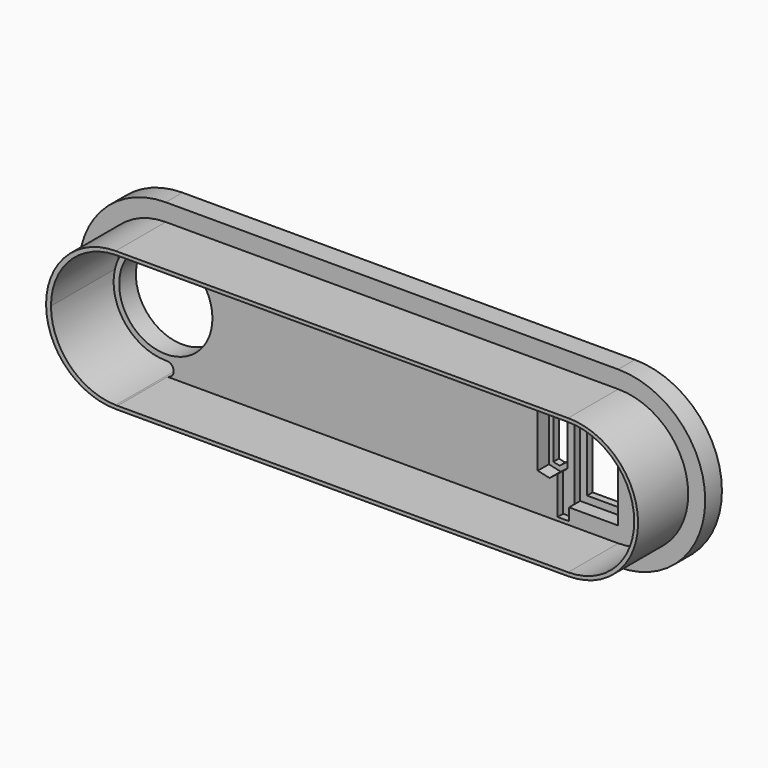
from build123d import *

# Parameters (mm, degrees)
F0_R     = 6.7
F1_DEPTH = 3
F2_DEPTH = 2
F0_W     = 5
F0_H     = 12.5
F3_DEPTH = 1
F4_DEPTH = 12


# Not quite as in the source:
# - ends of sketch curves that miss each other by under 0.0002 mm in the source are joined
# - a feature names something its author has since deleted; it is built from what else it names


with BuildPart() as f1:
    # F0 (on Front) → F1 (new body)
    with BuildSketch(Plane.XZ):
        with BuildLine():
            ThreePointArc((-65, 22), (-63.9934095883, 20.9934095883), (-65, 19.9868191765))
            ThreePointArc((-65, 19.9868191765), (-72.5, 12.4868191765), (-65, 4.9868191765))
            ThreePointArc((-65, 4.9868191765), (-63.8767141262, 4.1275392339), (-64.7360688632, 3.0043105795))
            Line((-64.7360688632, 3.0043105795), (0, 3))
            ThreePointArc((0, 3), (9.5, 12.5), (0, 22))
            Line((0, 22), (-65, 22))
        make_face()
        with Locations((-65, 12.4868191765)):
            Circle(F0_R, mode=Mode.SUBTRACT)
        Polygon((-7.0638221186, 19.7500795352), (-0.0638221186, 19.7500795352), (-0.0638221186, 5.2500795352), (-7.0638221186, 5.2500795352), (-7.0638221186, 3.5000024036), (-8.713822115, 3.5001122721), (-8.713822115, 8.9301122721), (-9.8584694148, 8.0498078222), (-11.5638221186, 8.4283766224), (-11.5638221186, 12.5000409694), (-11.5638221186, 16.5717053165), (-9.8584694148, 16.9502741166), (-8.713822115, 16.0699696667), (-8.713822115, 21.4999696667), (-7.0638221186, 21.5000795352), align=None, mode=Mode.SUBTRACT)
    extrude(amount=F1_DEPTH)



with BuildPart() as f1b:
    # F0 (on Front) → F1, piece 2 (new body)
    with BuildSketch(Plane.XZ):
        with BuildLine():
            Line((-65, 0), (0, 0))
            ThreePointArc((0, 0), (12.5, 12.5), (0, 25))
            Line((0, 25), (-65, 25))
            ThreePointArc((-65, 25), (-77.5, 12.5), (-65, 0))
        make_face()
        with BuildLine():
            ThreePointArc((-2.276e-07, 22.5000819376), (10.0557466602, 12.5000410832), (0, 2.5))
            Line((0, 2.5), (-65, 2.5))
            ThreePointArc((-65, 2.5), (-75.0000410826, 12.500040855), (-65.0000002276, 22.5000819376))
            Line((-65.0000002276, 22.5000819376), (-2.276e-07, 22.5000819376))
        make_face(mode=Mode.SUBTRACT)
    extrude(amount=F1_DEPTH)


with BuildPart() as f2:
    # F0 (on Front) → F2 (new body)
    with BuildSketch(Plane.XZ):
        Polygon((-7.0638221186, 12.5000795352), (-7.0638221186, 19.7500795352), (-7.0638221186, 21.5000795352), (-8.713822115, 21.4999696667), (-8.713822115, 16.0699696667), (-8.0638221186, 15.5700795352), (-8.0638221186, 9.4300024036), (-8.713822115, 8.9301122721), (-8.713822115, 3.5001122721), (-7.0638221186, 3.5000024036), (-7.0638221186, 5.2500024036), (-7.0638221186, 9.4300024036), align=None)
    extrude(amount=F2_DEPTH)


with BuildPart() as f3:
    # F0 (on Front) → F3 (new body)
    with BuildSketch(Plane.XZ):
        Polygon((-0.0638221186, 5.2500795352), (-0.0638221186, 19.7500795352), (-7.0638221186, 19.7500795352), (-7.0638221186, 12.5000795352), (-7.0638221186, 9.4300024036), (-7.0638221186, 5.2500795352), align=None)
        with Locations((-3.5638221186, 12.5000795352)):
            Rectangle(F0_W, F0_H, mode=Mode.SUBTRACT)
    extrude(amount=F3_DEPTH)


with BuildPart() as f3b:
    # F0 (on Front) → F3, piece 2 (new body)
    with BuildSketch(Plane.XZ):
        Polygon((-8.0638221186, 15.5700795352), (-8.713822115, 16.0699696667), (-9.8584694148, 16.9502741166), (-11.5638221186, 16.5717053165), (-11.5638221186, 12.5000409694), (-11.5638221186, 8.4283766224), (-9.8584694148, 8.0498078222), (-8.713822115, 8.9301122721), (-8.0638221186, 9.4300024036), align=None)
        Polygon((-10.0138316441, 16.249757261), (-8.7138221186, 15.2499696667), (-8.7138221186, 9.7501122721), (-10.0138316441, 8.7503246778), (-10.9138221186, 8.9501122721), (-10.9138221186, 9.7501122721), (-10.9138221186, 16.0499696667), align=None, mode=Mode.SUBTRACT)
    extrude(amount=F3_DEPTH)


with BuildPart() as f1_1:
    add(f1.part)

    add(f1b.part)  # F4 merges F1b
    # F0 (on Front) → F4 (join)
    with BuildSketch(Plane.XZ):
        with BuildLine():
            Line((-65, 2.5), (0, 2.5))
            ThreePointArc((0, 2.5), (10.0557466602, 12.5000410832), (-2.276e-07, 22.5000819376))
            Line((-2.276e-07, 22.5000819376), (-65.0000002276, 22.5000819376))
            ThreePointArc((-65.0000002276, 22.5000819376), (-75.0000410826, 12.500040855), (-65, 2.5))
        make_face()
        with BuildLine():
            ThreePointArc((-74.2972368995, 12.5000409694), (-71.5868031052, 19.1468457066), (-65, 22))
            Line((-65, 22), (0, 22))
            ThreePointArc((0, 22), (9.5, 12.5), (0, 3))
            Line((0, 3), (-64.7360688632, 3.0043105795))
            ThreePointArc((-64.7360688632, 3.0043105795), (-64.8680350139, 2.9955736674), (-65, 3.0043281539))
            ThreePointArc((-65, 3.0043281539), (-71.5853179489, 5.855965247), (-74.2972368995, 12.5000409694))
        make_face(mode=Mode.SUBTRACT)
    extrude(amount=F4_DEPTH)


solid = Compound([f2.part, f3.part, f3b.part, f1_1.part])
